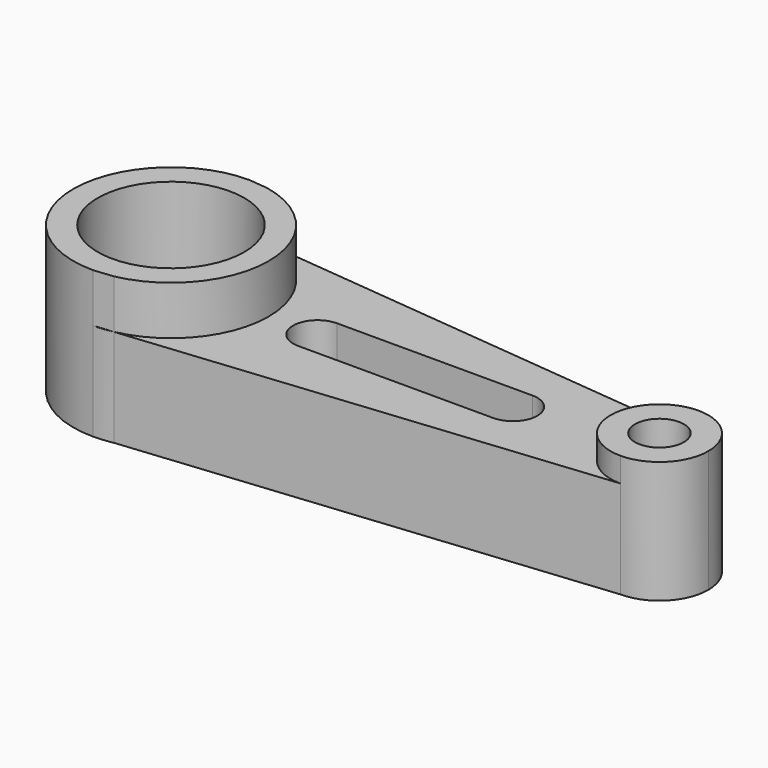
from build123d import *

# Parameters (mm, degrees)
F0_R     = 19.05
F1_DEPTH = 25.4
F2_DEPTH = 38.1
F0_R_2   = 6.35
F3_DEPTH = 31.75


with BuildPart() as f1:
    # F0 (on Top) → F1 (new body)
    with BuildSketch(Plane.XY):
        with BuildLine():
            Line((-58.4702970297, 24.897029703), (-63.5, 25.4))
            ThreePointArc((-63.5, 25.4), (-88.9, 0), (-63.5, -25.4))
            Line((-63.5, -25.4), (-58.4702970297, -24.897029703))
            ThreePointArc((-58.4702970297, -24.897029703), (-43.8414846002, -16.0842398725), (-38.1, 0))
            ThreePointArc((-38.1, 0), (-43.8414846002, 16.0842398725), (-58.4702970297, 24.897029703))
        make_face()
        with Locations((-63.5, 0)):
            Circle(F0_R, mode=Mode.SUBTRACT)
        with BuildLine():
            ThreePointArc((-58.4702970297, 24.897029703), (-60.9726055369, 25.2739446313), (-63.5, 25.4))
            Line((-63.5, 25.4), (-58.4702970297, 24.897029703))
        make_face()
        with BuildLine():
            Line((-58.4702970297, -24.897029703), (-63.5, -25.4))
            ThreePointArc((-63.5, -25.4), (-60.9726055369, -25.2739446313), (-58.4702970297, -24.897029703))
        make_face()
        with BuildLine():
            Line((63.5, 12.7), (-58.4702970297, 24.897029703))
            ThreePointArc((-58.4702970297, 24.897029703), (-43.8414846002, 16.0842398725), (-38.1, 0))
            ThreePointArc((-38.1, 0), (-43.8414846002, -16.0842398725), (-58.4702970297, -24.897029703))
            Line((-58.4702970297, -24.897029703), (63.5, -12.7))
            ThreePointArc((63.5, -12.7), (50.8, 0), (63.5, 12.7))
        make_face()
        with BuildLine():
            ThreePointArc((-25.4, -6.35), (-31.75, 0), (-25.4, 6.35))
            Line((-25.4, 6.35), (25.4, 6.35))
            ThreePointArc((25.4, 6.35), (31.75, 0), (25.4, -6.35))
            Line((25.4, -6.35), (-25.4, -6.35))
        make_face(mode=Mode.SUBTRACT)
    extrude(amount=F1_DEPTH)

    # F0 (on Top) → F2 (join)
    with BuildSketch(Plane.XY):
        with BuildLine():
            Line((-58.4702970297, 24.897029703), (-63.5, 25.4))
            ThreePointArc((-63.5, 25.4), (-88.9, 0), (-63.5, -25.4))
            Line((-63.5, -25.4), (-58.4702970297, -24.897029703))
            ThreePointArc((-58.4702970297, -24.897029703), (-43.8414846002, -16.0842398725), (-38.1, 0))
            ThreePointArc((-38.1, 0), (-43.8414846002, 16.0842398725), (-58.4702970297, 24.897029703))
        make_face()
        with Locations((-63.5, 0)):
            Circle(F0_R, mode=Mode.SUBTRACT)
    extrude(amount=F2_DEPTH)

    # F0 (on Top) → F3 (join)
    with BuildSketch(Plane.XY):
        with BuildLine():
            ThreePointArc((76.2, 0), (72.4802561211, 8.9802561211), (63.5, 12.7))
            ThreePointArc((63.5, 12.7), (50.8, 0), (63.5, -12.7))
            ThreePointArc((63.5, -12.7), (72.4802561211, -8.9802561211), (76.2, 0))
        make_face()
        with Locations((63.5, 0)):
            Circle(F0_R_2, mode=Mode.SUBTRACT)
    extrude(amount=F3_DEPTH)


solid = f1.part
